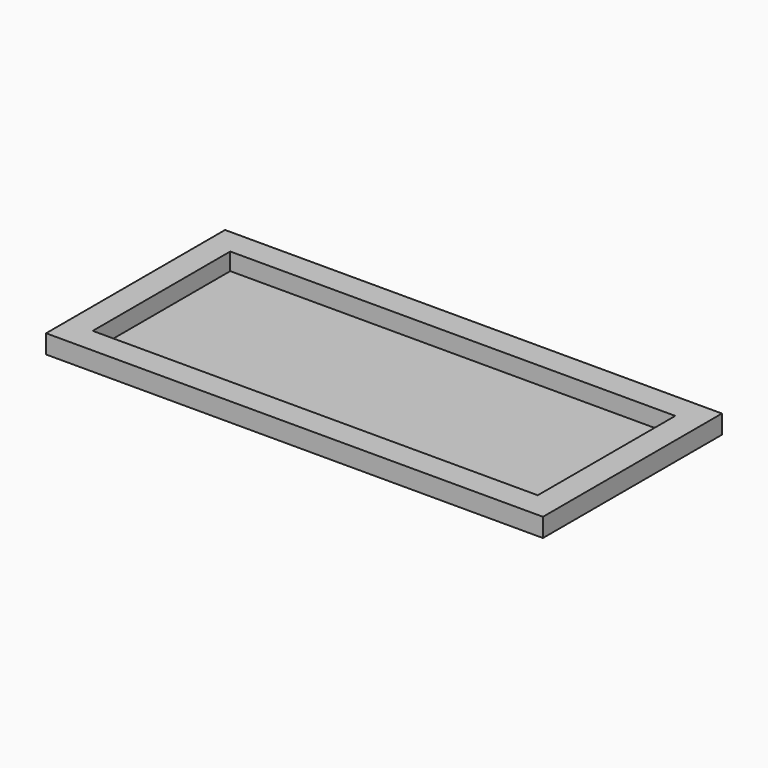
from build123d import *

# Parameters (mm, degrees)
F0_W     = 311.15
F0_H     = 121.4
F0_R     = 2.5
F0_R_2   = 2
F1_DEPTH = 13
F2_T     = -1
F4_DEPTH = 17
F5_DEPTH = 17
F6_DEPTH = 17
F7_DEPTH = 17


# Not quite as in the source:
# - the program builds the solid bodies; features that only make, move or delete a surface that nothing else refers to are left out


with BuildPart() as f1:
    # F0 (on Top) → F1 (new body)
    with BuildSketch(Plane.XY):
        with Locations((6.6334828734, -24.2652736852)):
            Rectangle(F0_W, F0_H)
        with Locations((-116.9415171266, -32.9652736852)):
            Circle(F0_R, mode=Mode.SUBTRACT)
        with Locations((-61.4415171266, -23.5952736852)):
            Circle(F0_R_2, mode=Mode.SUBTRACT)
        with Locations((74.7084828734, -23.5652736852)):
            Circle(F0_R_2, mode=Mode.SUBTRACT)
        with Locations((114.5584828734, -13.7852736852)):
            Circle(F0_R, mode=Mode.SUBTRACT)
        with Locations((-116.9415171266, -32.9652736852)):
            Circle(F0_R)
        with Locations((114.5584828734, -13.7852736852)):
            Circle(F0_R)
        with Locations((-61.4415171266, -23.5952736852)):
            Circle(F0_R_2)
        with Locations((74.7084828734, -23.5652736852)):
            Circle(F0_R_2)
    extrude(amount=F1_DEPTH)

    # F2
    f2_openings = [f1.faces().sort_by_distance(p)[0] for p in [
        (6.633483, -24.265274, 13),
    ]]
    offset(amount=F2_T, openings=f2_openings)

    # F4 (add): a face of the model
    f4_faces = [f1.faces().sort_by_distance(p)[0] for p in [
        (6.6334828734, -84.9652736852, 6.5),
    ]]
    extrude(f4_faces, amount=F4_DEPTH)

    # F5 (add): a face of the model
    f5_faces = [f1.faces().sort_by_distance(p)[0] for p in [
        (-148.9415171266, -32.7652736852, 6.5),
    ]]
    extrude(f5_faces, amount=F5_DEPTH)

    # F6 (add): a face of the model
    f6_faces = [f1.faces().sort_by_distance(p)[0] for p in [
        (162.2084828734, -32.7652736852, 6.5),
    ]]
    extrude(f6_faces, amount=F6_DEPTH)

    # F7 (add): a face of the model
    f7_faces = [f1.faces().sort_by_distance(p)[0] for p in [
        (6.6334828734, 36.4347263148, 6.5),
    ]]
    extrude(f7_faces, amount=F7_DEPTH)


solid = f1.part
